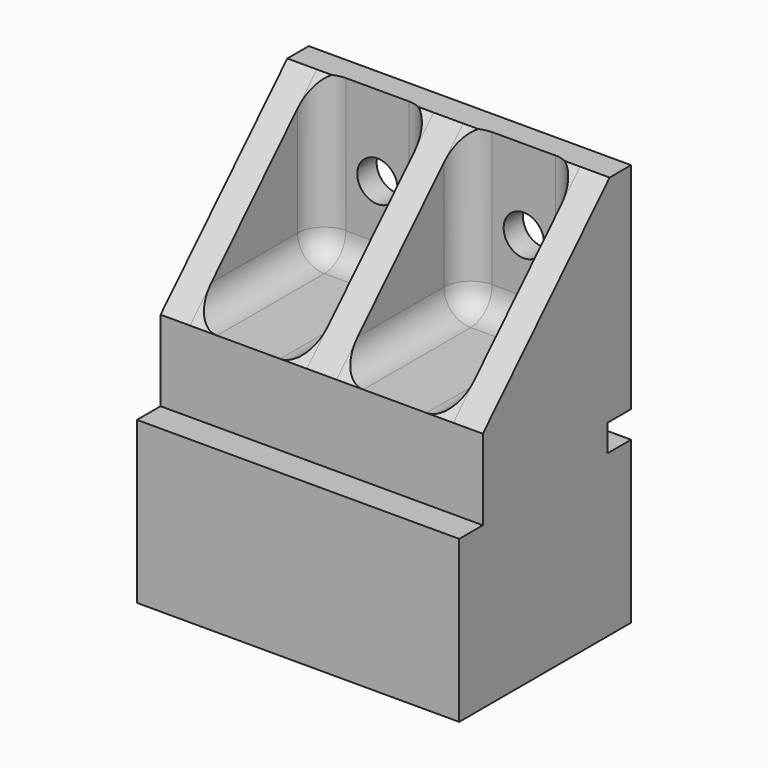
from build123d import *

# Parameters (mm, degrees)
F1_DEPTH     = 38.1
F2_W         = 13.81125
F2_H         = 19.05
F3_DEPTH     = 19.05
F4_T1_DEPTH  = 7.46125
F4_T3_DEPTH  = 7.46125
F4_S7_W      = 3.175
F4_S7_H      = 3.175
F4_T8_DEPTH  = 3.175
F4_S13_W     = 3.175
F4_S13_H     = 3.175
F4_T14_DEPTH = 3.175
F4_S19_W     = 3.175
F4_S19_H     = 3.175
F4_T20_DEPTH = 3.175
F4_S25_W     = 3.175
F4_S25_H     = 3.175
F4_T26_DEPTH = 3.175
F4_T32_DEPTH = 15.875
F4_T37_DEPTH = 15.875
F4_T42_DEPTH = 15.875
F4_T47_DEPTH = 15.875
F4_T52_DEPTH = 15.875
F4_T57_DEPTH = 15.875
F4_T62_DEPTH = 15.875
F4_T67_DEPTH = 15.875
F6_DEPTH     = 2.8585


# Not quite as in the source:
# - a fillet or chamfer that OpenCascade refuses, or shapes differently, is made with other operations: its cross-section is extruded or revolved along the edge and cut away or added


with BuildPart() as f1:
    # F0 (on Right) → F1 (new body)
    with BuildSketch(Plane.YZ):
        Polygon((0, 19.05), (0, 0), (25.4, 0), (25.4, 19.05), (21.9075, 19.05), (21.9075, 22.225), (25.4, 22.225), (25.4, 47.625), (22.225, 47.625), (22.225, 28.575), (3.4925, 28.575), (3.4925, 19.05), align=None)
        Polygon((22.225, 47.625), (3.4925, 28.575), (22.225, 28.575), align=None)
    extrude(amount=F1_DEPTH)

    # F2 (on face) → F3 (cut)
    with BuildSketch(Plane.XZ.offset(-3.4925)):
        with Locations((27.701875, 38.1)):
            Rectangle(F2_W, F2_H)
        with Locations((10.398125, 38.1)):
            Rectangle(F2_W, F2_H)
    extrude(amount=-F3_DEPTH, mode=Mode.SUBTRACT)

    # F4: fillet of radius 3.175 on 10 edges, made by hand

    # F4_s2 → F4_t1 (join)
    with BuildSketch(Plane.YZ.offset(6.6675)):
        with BuildLine():
            ThreePointArc((19.3675, 28.575), (21.6125640303, 29.5049359697), (22.5425, 31.75))
            Line((22.5425, 31.75), (22.5425, 28.575))
            Line((22.5425, 28.575), (19.3675, 28.575))
        make_face()
    extrude(amount=F4_T1_DEPTH)

    # F4_s4 → F4_t3 (join)
    with BuildSketch(Plane.YZ.offset(23.97125)):
        with BuildLine():
            ThreePointArc((19.3675, 28.575), (21.6125640303, 29.5049359697), (22.5425, 31.75))
            Line((22.5425, 31.75), (22.5425, 28.575))
            Line((22.5425, 28.575), (19.3675, 28.575))
        make_face()
    extrude(amount=F4_T3_DEPTH)


with BuildPart() as f4_tool6:
    # F4_s7 → F4_t8 (new body)
    with BuildSketch(Plane.YZ.offset(6.6675)):
        with Locations((20.955, 30.1625)):
            Rectangle(F4_S7_W, F4_S7_H)
    extrude(amount=-F4_T8_DEPTH)

    # F4_s9 → F4_t10 (revolve, cut)
    with BuildSketch(Plane(origin=(6.6675, 19.3675, 31.75), x_dir=(0, -0.7071067812, 0.7071067812), z_dir=(0, -0.7071067812, -0.7071067812))):
        with BuildLine():
            ThreePointArc((0, -3.175), (3.175, 0), (0, 3.175))
            Line((0, 3.175), (0, -3.175))
        make_face()
    revolve(axis=Axis((6.6675, 19.3675, 31.75), (-1, 0, 0)), mode=Mode.SUBTRACT)


with BuildPart() as f1_1:
    add(f1.part)

    # F4_t5: union F4_tool6
    add(f4_tool6.part)


with BuildPart() as f4_tool12:
    # F4_s13 → F4_t14 (new body)
    with BuildSketch(Plane.XZ.offset(-19.3675)):
        with Locations((15.71625, 30.1625)):
            Rectangle(F4_S13_W, F4_S13_H)
    extrude(amount=-F4_T14_DEPTH)

    # F4_s15 → F4_t16 (revolve, cut)
    with BuildSketch(Plane(origin=(14.12875, 19.3675, 31.75), x_dir=(-0.7071067812, 0, 0.7071067812), z_dir=(-0.7071067812, 0, -0.7071067812))):
        with BuildLine():
            ThreePointArc((0, -3.175), (3.175, 0), (0, 3.175))
            Line((0, 3.175), (0, -3.175))
        make_face()
    revolve(axis=Axis((14.12875, 19.3675, 31.75), (0, 1, 0)), mode=Mode.SUBTRACT)


with BuildPart() as f1_2:
    add(f1_1.part)

    # F4_t11: union F4_tool12
    add(f4_tool12.part)


with BuildPart() as f4_tool18:
    # F4_s19 → F4_t20 (new body)
    with BuildSketch(Plane.XY.offset(31.75)):
        with Locations((22.38375, 20.955)):
            Rectangle(F4_S19_W, F4_S19_H)
    extrude(amount=-F4_T20_DEPTH)

    # F4_s21 → F4_t22 (revolve, cut)
    with BuildSketch(Plane(origin=(23.97125, 19.3675, 31.75), x_dir=(0.7071067812, -0.7071067812, 0), z_dir=(0.7071067812, 0.7071067812, 0))):
        with BuildLine():
            ThreePointArc((0, -3.175), (3.175, 0), (0, 3.175))
            Line((0, 3.175), (0, -3.175))
        make_face()
    revolve(axis=Axis((23.97125, 19.3675, 31.75), (0, 0, -1)), mode=Mode.SUBTRACT)


with BuildPart() as f1_3:
    add(f1_2.part)

    # F4_t17: union F4_tool18
    add(f4_tool18.part)


with BuildPart() as f4_tool24:
    # F4_s25 → F4_t26 (new body)
    with BuildSketch(Plane.XY.offset(31.75)):
        with Locations((33.02, 20.955)):
            Rectangle(F4_S25_W, F4_S25_H)
    extrude(amount=-F4_T26_DEPTH)

    # F4_s27 → F4_t28 (revolve, cut)
    with BuildSketch(Plane(origin=(31.4325, 19.3675, 31.75), x_dir=(-0.7071067812, -0.7071067812, 0), z_dir=(0.7071067812, -0.7071067812, 0))):
        with BuildLine():
            ThreePointArc((0, -3.175), (3.175, 0), (0, 3.175))
            Line((0, 3.175), (0, -3.175))
        make_face()
    revolve(axis=Axis((31.4325, 19.3675, 31.75), (0, 0, -1)), mode=Mode.SUBTRACT)


with BuildPart() as f1_4:
    add(f1_3.part)

    # F4_t23: union F4_tool24
    add(f4_tool24.part)


with BuildPart() as f4_tool30:
    # F4_s31 → F4_t32 (new body)
    with BuildSketch(Plane.XY.offset(47.625)):
        with BuildLine():
            ThreePointArc((20.79625, 19.3675), (21.7261859697, 21.6125640303), (23.97125, 22.5425))
            Line((23.97125, 22.5425), (20.79625, 22.5425))
            Line((20.79625, 22.5425), (20.79625, 19.3675))
        make_face()
    extrude(amount=-F4_T32_DEPTH)

    split(bisect_by=Plane(origin=(0, -12.5098856094, 12.3013875159), x_dir=(1, 0, 0), z_dir=(0, 0.7130236798, -0.7011399518)), keep=Keep.TOP)


with BuildPart() as f1_5:
    add(f1_4.part)

    # F4_t29: union F4_tool30
    add(f4_tool30.part)


with BuildPart() as f4_tool35:
    # F4_s36 → F4_t37 (new body)
    with BuildSketch(Plane.XZ.offset(-3.4925)):
        with BuildLine():
            ThreePointArc((23.97125, 28.575), (21.7261859697, 29.5049359697), (20.79625, 31.75))
            Line((20.79625, 31.75), (20.79625, 28.575))
            Line((20.79625, 28.575), (23.97125, 28.575))
        make_face()
    extrude(amount=-F4_T37_DEPTH)

    split(bisect_by=Plane(origin=(0, -12.5098856094, 12.3013875159), x_dir=(1, 0, 0), z_dir=(0, 0.7130236798, -0.7011399518)), keep=Keep.TOP)


with BuildPart() as f1_6:
    add(f1_5.part)

    # F4_t34: union F4_tool35
    add(f4_tool35.part)


with BuildPart() as f4_tool40:
    # F4_s41 → F4_t42 (new body)
    with BuildSketch(Plane.XY.offset(47.625)):
        with BuildLine():
            ThreePointArc((3.4925, 19.3675), (4.4224359697, 21.6125640303), (6.6675, 22.5425))
            Line((6.6675, 22.5425), (3.4925, 22.5425))
            Line((3.4925, 22.5425), (3.4925, 19.3675))
        make_face()
    extrude(amount=-F4_T42_DEPTH)

    split(bisect_by=Plane(origin=(0, -12.5098856094, 12.3013875159), x_dir=(1, 0, 0), z_dir=(0, 0.7130236798, -0.7011399518)), keep=Keep.TOP)


with BuildPart() as f1_7:
    add(f1_6.part)

    # F4_t39: union F4_tool40
    add(f4_tool40.part)


with BuildPart() as f4_tool45:
    # F4_s46 → F4_t47 (new body)
    with BuildSketch(Plane.XZ.offset(-3.4925)):
        with BuildLine():
            ThreePointArc((6.6675, 28.575), (4.4224359697, 29.5049359697), (3.4925, 31.75))
            Line((3.4925, 31.75), (3.4925, 28.575))
            Line((3.4925, 28.575), (6.6675, 28.575))
        make_face()
    extrude(amount=-F4_T47_DEPTH)

    split(bisect_by=Plane(origin=(0, -12.5098856094, 12.3013875159), x_dir=(1, 0, 0), z_dir=(0, 0.7130236798, -0.7011399518)), keep=Keep.TOP)


with BuildPart() as f1_8:
    add(f1_7.part)

    # F4_t44: union F4_tool45
    add(f4_tool45.part)


with BuildPart() as f4_tool50:
    # F4_s51 → F4_t52 (new body)
    with BuildSketch(Plane.XZ.offset(-3.4925)):
        with BuildLine():
            ThreePointArc((31.4325, 28.575), (33.6775640303, 29.5049359697), (34.6075, 31.75))
            Line((34.6075, 31.75), (34.6075, 28.575))
            Line((34.6075, 28.575), (31.4325, 28.575))
        make_face()
    extrude(amount=-F4_T52_DEPTH)

    split(bisect_by=Plane(origin=(0, -12.5098856094, 12.3013875159), x_dir=(1, 0, 0), z_dir=(0, 0.7130236798, -0.7011399518)), keep=Keep.TOP)


with BuildPart() as f1_9:
    add(f1_8.part)

    # F4_t49: union F4_tool50
    add(f4_tool50.part)


with BuildPart() as f4_tool55:
    # F4_s56 → F4_t57 (new body)
    with BuildSketch(Plane.XY.offset(31.75)):
        with BuildLine():
            ThreePointArc((31.4325, 22.5425), (33.6775640303, 21.6125640303), (34.6075, 19.3675))
            Line((34.6075, 19.3675), (34.6075, 22.5425))
            Line((34.6075, 22.5425), (31.4325, 22.5425))
        make_face()
    extrude(amount=F4_T57_DEPTH)

    split(bisect_by=Plane(origin=(0, -12.5098856094, 12.3013875159), x_dir=(1, 0, 0), z_dir=(0, 0.7130236798, -0.7011399518)), keep=Keep.TOP)


with BuildPart() as f1_10:
    add(f1_9.part)

    # F4_t54: union F4_tool55
    add(f4_tool55.part)


with BuildPart() as f4_tool60:
    # F4_s61 → F4_t62 (new body)
    with BuildSketch(Plane.XZ.offset(-3.4925)):
        with BuildLine():
            ThreePointArc((14.12875, 28.575), (16.3738140303, 29.5049359697), (17.30375, 31.75))
            Line((17.30375, 31.75), (17.30375, 28.575))
            Line((17.30375, 28.575), (14.12875, 28.575))
        make_face()
    extrude(amount=-F4_T62_DEPTH)

    split(bisect_by=Plane(origin=(0, -12.5098856094, 12.3013875159), x_dir=(1, 0, 0), z_dir=(0, 0.7130236798, -0.7011399518)), keep=Keep.TOP)


with BuildPart() as f1_11:
    add(f1_10.part)

    # F4_t59: union F4_tool60
    add(f4_tool60.part)


with BuildPart() as f4_tool65:
    # F4_s66 → F4_t67 (new body)
    with BuildSketch(Plane.XY.offset(31.75)):
        with BuildLine():
            ThreePointArc((14.12875, 22.5425), (16.3738140303, 21.6125640303), (17.30375, 19.3675))
            Line((17.30375, 19.3675), (17.30375, 22.5425))
            Line((17.30375, 22.5425), (14.12875, 22.5425))
        make_face()
    extrude(amount=F4_T67_DEPTH)

    split(bisect_by=Plane(origin=(0, -12.5098856094, 12.3013875159), x_dir=(1, 0, 0), z_dir=(0, 0.7130236798, -0.7011399518)), keep=Keep.TOP)


with BuildPart() as f1_12:
    add(f1_11.part)

    # F4_t64: union F4_tool65
    add(f4_tool65.part)

    # F5 (on face) → F6 (cut, through all)
    with BuildSketch(Plane.XZ.offset(-22.5425)):
        with BuildLine():
            ThreePointArc((10.398125, 35.71875), (12.0819230227, 36.4162019773), (12.779375, 38.1))
            ThreePointArc((12.779375, 38.1), (8.7143269773, 39.7837980227), (10.398125, 35.71875))
        make_face()
        with BuildLine():
            ThreePointArc((27.701875, 35.71875), (29.3856730227, 36.4162019773), (30.083125, 38.1))
            ThreePointArc((30.083125, 38.1), (26.0180769773, 39.7837980227), (27.701875, 35.71875))
        make_face()
    extrude(amount=-F6_DEPTH, mode=Mode.SUBTRACT)


solid = f1_12.part
